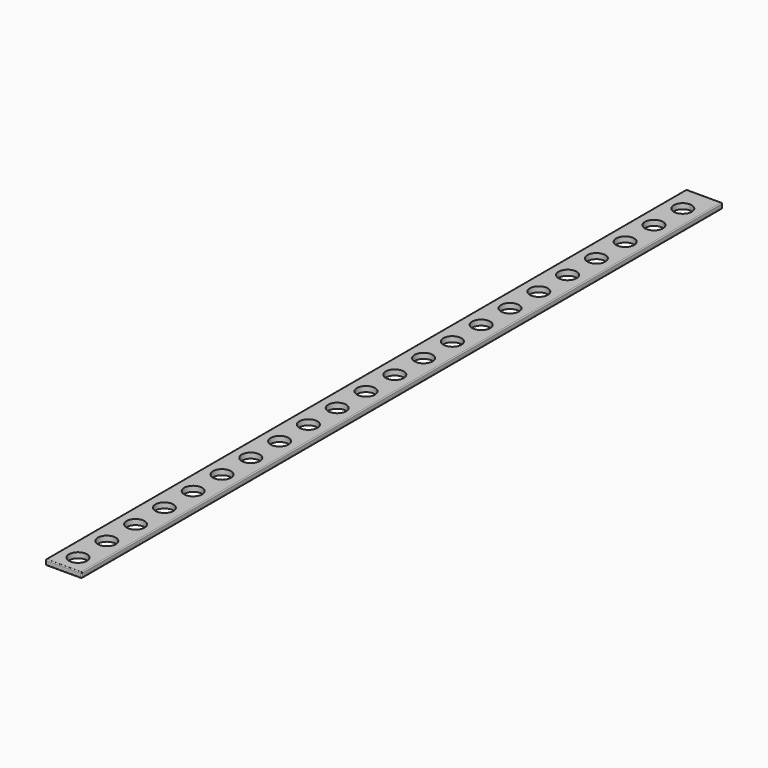
from build123d import *

# Parameters (mm, degrees)
F0_W     = 20
F0_H     = 3
F1_DEPTH = 250
F3_DEPTH = 10
F2_R     = 5
F4_DEPTH = 3
F5_R     = 0.5
F7_DEPTH = 25
F8_R     = 0.5


with BuildPart() as f1:
    # F0 (on Front) → F1 (new body, symmetric)
    with BuildSketch(Plane.XZ):
        Rectangle(F0_W, F0_H)
    extrude(amount=F1_DEPTH, both=True)

    # F3 (add): a face of the model
    f3_faces = [f1.faces().sort_by_distance(p)[0] for p in [
        (0, 250, 0),
    ]]
    extrude(f3_faces, amount=F3_DEPTH)

    # F2 (on face) → F4 (cut)
    with BuildSketch(Plane.XY.offset(1.5)):
        with BuildLine():
            ThreePointArc((5, -215), (-3.5355339059, -211.4644660941), (0, -220))
            ThreePointArc((0, -220), (3.5355339059, -218.5355339059), (5, -215))
        make_face()
        with BuildLine():
            ThreePointArc((0, -230), (-5, -235), (0, -240))
            ThreePointArc((0, -240), (3.5355339059, -238.5355339059), (5, -235))
            ThreePointArc((5, -235), (3.5355339059, -231.4644660941), (0, -230))
        make_face()
        with BuildLine():
            ThreePointArc((5, 245), (3.5355339059, 248.5355339059), (0, 250))
            ThreePointArc((0, 250), (-3.5355339059, 241.4644660941), (5, 245))
        make_face()
        with Locations((0, -195)):
            Circle(F2_R)
        with Locations((0, -175)):
            Circle(F2_R)
        with Locations((0, -155)):
            Circle(F2_R)
        with Locations((0, -135)):
            Circle(F2_R)
        with Locations((0, -115)):
            Circle(F2_R)
        with Locations((0, -95)):
            Circle(F2_R)
        with Locations((0, -75)):
            Circle(F2_R)
        with Locations((0, -55)):
            Circle(F2_R)
        with Locations((0, -35)):
            Circle(F2_R)
        with Locations((0, -15)):
            Circle(F2_R)
        with Locations((0, 5)):
            Circle(F2_R)
        with Locations((0, 25)):
            Circle(F2_R)
        with Locations((0, 45)):
            Circle(F2_R)
        with Locations((0, 65)):
            Circle(F2_R)
        with Locations((0, 85)):
            Circle(F2_R)
        with Locations((0, 105)):
            Circle(F2_R)
        with Locations((0, 125)):
            Circle(F2_R)
        with Locations((0, 145)):
            Circle(F2_R)
        with Locations((0, 165)):
            Circle(F2_R)
        with Locations((0, 185)):
            Circle(F2_R)
        with Locations((0, 205)):
            Circle(F2_R)
        with Locations((0, 225)):
            Circle(F2_R)
    extrude(amount=-F4_DEPTH, mode=Mode.SUBTRACT)

    # F5
    f5_edges = [f1.edges().sort_by_distance(p)[0] for p in [
        (10, -250, 0),
        (10, 5, -1.5),
        (10, 260, 0),
        (10, 5, 1.5),
        (0, -250, 1.5),
        (-10, -250, 0),
        (0, -250, -1.5),
        (-10, 5, 1.5),
        (0, 260, 1.5),
        (-10, 260, 0),
        (0, 260, -1.5),
    ]]
    fillet(f5_edges, radius=F5_R)

    # F6 (on face) → F7 (cut)
    with BuildSketch(Plane(origin=(0, 0, -1.5), x_dir=(1, 0, 0), z_dir=(0, 0, -1))):
        Polygon((0, 185), (16.080936417, 185), (32.4585177004, 259.3803107738), (-14.6508449689, 254.37900424), (-14.6508449689, 185), align=None)
    extrude(amount=-F7_DEPTH, mode=Mode.SUBTRACT)

    # F8
    f8_edges = [f1.edges().sort_by_distance(p)[0] for p in [
        (9.853553, -185, -1.353553),
        (10, -185, 0),
        (9.853553, -185, 1.353553),
        (0, -185, 1.5),
        (-9.853553, -185, 1.353553),
        (-10, -185, -0.25),
        (-0.25, -185, -1.5),
    ]]
    fillet(f8_edges, radius=F8_R)


solid = f1.part
